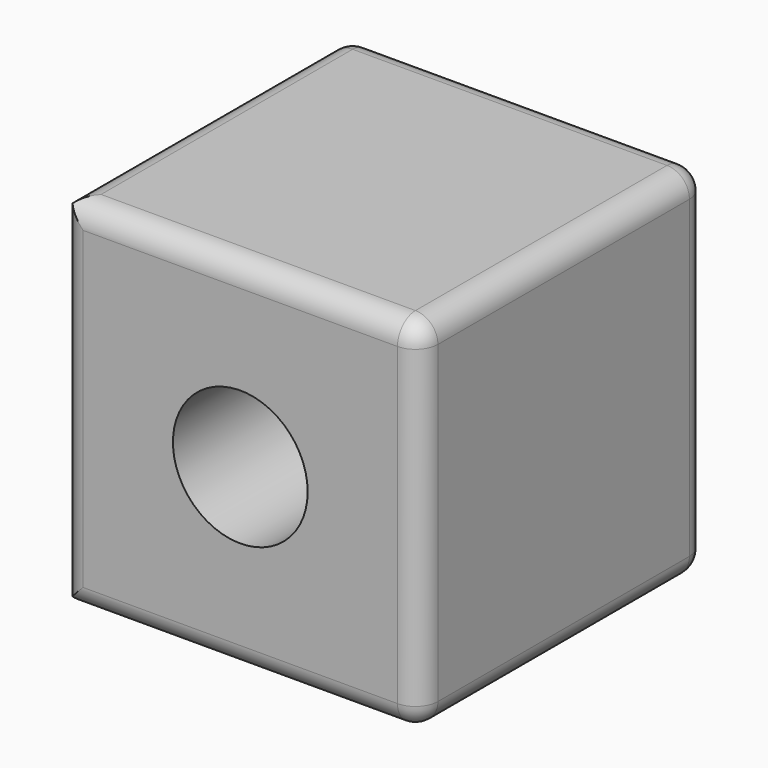
from build123d import *

# Parameters (mm, degrees)
F0_W         = 80
F0_H         = 80
F1_DEPTH     = 40
F2_R         = 5
F3_T1_DEPTH  = 82.5
F3_S5_W      = 5.1
F3_S5_H      = 5.1
F3_T6_DEPTH  = 5.1
F3_S11_W     = 5.1
F3_S11_H     = 5.1
F3_T12_DEPTH = 5.1
F4_R         = 15
F5_DEPTH     = 80.001


# Not quite as in the source:
# - a fillet or chamfer that OpenCascade refuses, or shapes differently, is made with other operations: its cross-section is extruded or revolved along the edge and cut away or added


with BuildPart() as f1:
    # F0 (on Top) → F1 (new body, symmetric)
    with BuildSketch(Plane.XY):
        Rectangle(F0_W, F0_H)
    extrude(amount=F1_DEPTH, both=True)

    # F2
    f2_edges = [f1.edges().sort_by_distance(p)[0] for p in [
        (0, -40, 40),
        (-40, -40, 0),
        (40, -40, 0),
        (0, -40, -40),
        (40, 0, 40),
        (40, 40, 0),
        (40, 0, -40),
        (0, 40, 40),
        (-40, 40, 0),
        (0, 40, -40),
    ]]
    fillet(f2_edges, radius=F2_R)

    # F3: fillet of radius 5 on 6 edges, made by hand

    # F3_s2 → F3_t1 (cut)
    with BuildSketch(Plane.XZ.offset(-35)):
        with BuildLine():
            ThreePointArc((-35, 40), (-38.5355339059, 38.5355339059), (-40, 35))
            Line((-40, 35), (-40, 40))
            Line((-40, 40), (-35, 40))
        make_face()
        with BuildLine():
            ThreePointArc((-35, -40), (-38.5355339059, -38.5355339059), (-40, -35))
            Line((-40, -35), (-40, -40))
            Line((-40, -40), (-35, -40))
        make_face()
    extrude(amount=F3_T1_DEPTH, mode=Mode.SUBTRACT)


with BuildPart() as f3_tool4:
    # F3_s5 → F3_t6 (new body)
    with BuildSketch(Plane.XY.offset(-35)):
        with Locations((-37.55, 37.55)):
            Rectangle(F3_S5_W, F3_S5_H)
    extrude(amount=-F3_T6_DEPTH)

    # F3_s7 → F3_t8 (revolve, cut)
    with BuildSketch(Plane(origin=(-35, 35, -35), x_dir=(0.7071067812, -0.7071067812, 0), z_dir=(0.7071067812, 0.7071067812, 0))):
        with BuildLine():
            ThreePointArc((0, -5), (5, 0), (0, 5))
            Line((0, 5), (0, -5))
        make_face()
    revolve(axis=Axis((-35, 35, -35), (0, 0, -1)), mode=Mode.SUBTRACT)


with BuildPart() as f1_1:
    add(f1.part)

    # F3_t3: cut F3_tool4
    add(f3_tool4.part, mode=Mode.SUBTRACT)


with BuildPart() as f3_tool10:
    # F3_s11 → F3_t12 (new body)
    with BuildSketch(Plane.XY.offset(35)):
        with Locations((-37.55, 37.55)):
            Rectangle(F3_S11_W, F3_S11_H)
    extrude(amount=F3_T12_DEPTH)

    # F3_s13 → F3_t14 (revolve, cut)
    with BuildSketch(Plane(origin=(-35, 35, 35), x_dir=(0.7071067812, -0.7071067812, 0), z_dir=(-0.7071067812, -0.7071067812, 0))):
        with BuildLine():
            ThreePointArc((0, -5), (5, 0), (0, 5))
            Line((0, 5), (0, -5))
        make_face()
    revolve(axis=Axis((-35, 35, 35), (0, 0, 1)), mode=Mode.SUBTRACT)


with BuildPart() as f1_2:
    add(f1_1.part)

    # F3_t9: cut F3_tool10
    add(f3_tool10.part, mode=Mode.SUBTRACT)

    # F4 (on face) → F5 (cut, through all)
    with BuildSketch(Plane.XZ.offset(40)):
        Circle(F4_R)
    extrude(amount=-F5_DEPTH, mode=Mode.SUBTRACT)


solid = f1_2.part
